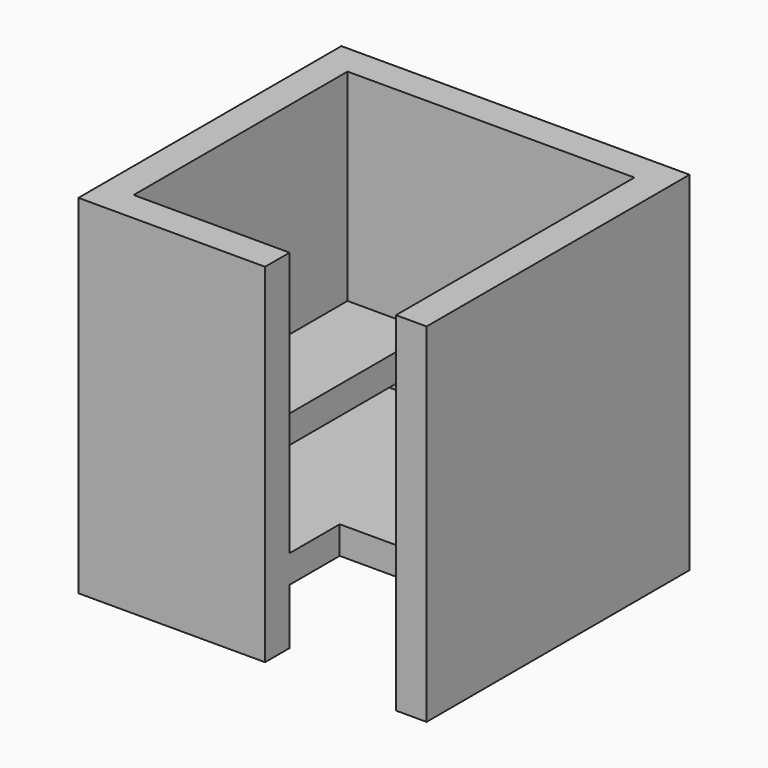
from build123d import *

# Parameters (mm, degrees)
F1_DEPTH = 2500
F2_W     = 2060
F2_H     = 200
F3_DEPTH = 1920
F4_W     = 1920
F4_H     = 200
F5_DEPTH = 600
F6_R     = 200
F7_DEPTH = 465
F8_W     = 940
F8_H     = 450
F9_DEPTH = 200


# Not quite as in the source:
# - the program builds the solid bodies; features that only make, move or delete a surface that nothing else refers to are left out


with BuildPart() as f1:
    # F0 (on Top) → F1 (new body)
    with BuildSketch(Plane.XY):
        Polygon((-1030, 960), (1030, 960), (1030, -960), (1030, -1180), (1250, -1180), (1250, 1180), (-1250, 1180), (-1250, -1180), (90, -1180), (90, -960), (-1030, -960), align=None)
    extrude(amount=F1_DEPTH)

    # F2 (on face) → F3 (join)
    with BuildSketch(Plane.XZ.offset(-960)):
        with Locations((0, 500)):
            Rectangle(F2_W, F2_H)
    extrude(amount=F3_DEPTH)

    # F4 (on face) → F5 (join)
    with BuildSketch(Plane.YZ.offset(-1030)):
        with Locations((0, 950)):
            Rectangle(F4_W, F4_H)
    extrude(amount=F5_DEPTH)

    # F6 (on face) → F7 (join)
    with BuildSketch(Plane.XY.offset(600)):
        with Locations((730, 660)):
            Circle(F6_R)
    extrude(amount=F7_DEPTH)

    # F8 (on face) → F9 (cut, through all)
    with BuildSketch(Plane.XY.offset(600)):
        with Locations((560, -735)):
            Rectangle(F8_W, F8_H)
    extrude(amount=-F9_DEPTH, mode=Mode.SUBTRACT)


solid = f1.part
